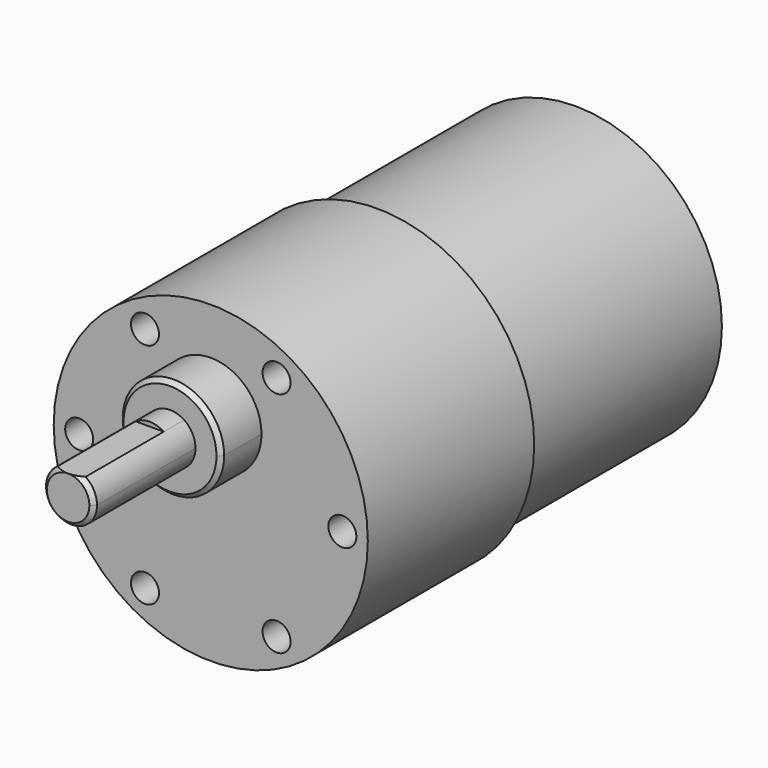
from build123d import *

# Parameters (mm, degrees)
F0_R      = 18.5
F0_R_2    = 17.25
F0_R_3    = 16.7
F0_R_4    = 4.1
F1_DEPTH  = 24.5
F2_DEPTH  = 53.7
F3_R      = 16.7
F3_R_2    = 4.1
F4_DEPTH  = 1
F5_DEPTH  = 1.2
F7_D      = 3.3
F7_DEPTH  = 4
F7_TIP    = 0.9914200214
F8_DEPTH  = 21
F9_DEPTH  = 6
F11_DEPTH = 12
F13_SIZE  = 0.49999


# Not quite as in the source:
# - a fillet or chamfer is up to 0.001 mm smaller than in the source, because OpenCascade refuses the exact size
# - a feature of the source that left no trace in its solid (it failed there, or was rolled back) is left out
# - a feature names something its author has since deleted; it is built from what else it names


with BuildPart() as f1:
    # F0 (on Front) → F1 (new body)
    with BuildSketch(Plane.XZ):
        Circle(F0_R)
        Circle(F0_R_2, mode=Mode.SUBTRACT)
        Circle(F0_R_2)
        Circle(F0_R_3, mode=Mode.SUBTRACT)
        Circle(F0_R_3)
        Circle(F0_R_4, mode=Mode.SUBTRACT)
        Circle(F0_R_4)
    extrude(amount=-F1_DEPTH)

    # F0 (on Front) → F2 (join)
    with BuildSketch(Plane.XZ):
        Circle(F0_R_2)
        Circle(F0_R_3, mode=Mode.SUBTRACT)
        Circle(F0_R_3)
        Circle(F0_R_4, mode=Mode.SUBTRACT)
        Circle(F0_R_4)
    extrude(amount=-F2_DEPTH)

    # F3 (on face) → F4 (cut)
    with BuildSketch(Plane(origin=(0, 53.7, 0), x_dir=(-1, 0, 0), z_dir=(0, 1, 0))):
        Circle(F3_R)
        Circle(F3_R_2, mode=Mode.SUBTRACT)
    extrude(amount=-F4_DEPTH, mode=Mode.SUBTRACT)

    # F5 (add): a face of the model
    f5_faces = [f1.faces().sort_by_distance(p)[0] for p in [
        (0, 53.7, 0),
    ]]
    extrude(f5_faces, amount=F5_DEPTH)

    # F7
    with Locations(Plane.XZ):
        with Locations((7.75, 13.4233937587), (15.5, 0), (7.75, -13.4233937587), (-7.75, -13.4233937587), (-15.5, 0), (-7.75, 13.4233937587)):
            Hole(F7_D / 2, depth=F7_DEPTH)
            with Locations((0, 0, -(F7_DEPTH + F7_TIP / 2))):  # 118° drill point
                Cone(0, F7_D / 2, F7_TIP, mode=Mode.SUBTRACT)

    # F6 (on face) → F8 (join)
    with BuildSketch(Plane.XZ):
        with BuildLine():
            ThreePointArc((0.5863406929, 4.0578571429), (0, 4.1), (-0.5863406929, 4.0578571429))
            ThreePointArc((-0.5863406929, 4.0578571429), (0, 4), (0.5863406929, 4.0578571429))
        make_face()
        with BuildLine():
            ThreePointArc((-1.6583123952, 9.5), (-2.9434412837, 6.4202126173), (-0.5863406929, 4.0578571429))
            ThreePointArc((-0.5863406929, 4.0578571429), (0, 4.1), (0.5863406929, 4.0578571429))
            ThreePointArc((0.5863406929, 4.0578571429), (2.3193772956, 5.0972417493), (3, 7))
            ThreePointArc((3, 7), (2.6433820369, 8.4186371655), (1.6583123952, 9.5))
            Line((1.6583123952, 9.5), (-1.6583123952, 9.5))
        make_face()
        with BuildLine():
            ThreePointArc((1.6583123952, 9.5), (0, 10), (-1.6583123952, 9.5))
            Line((-1.6583123952, 9.5), (1.6583123952, 9.5))
        make_face()
    extrude(amount=F8_DEPTH)

    # F6 (on face) → F9 (join)
    with BuildSketch(Plane.XZ):
        with BuildLine():
            ThreePointArc((-0.5863406929, 4.0578571429), (-2.2505108877, 3.4271271853), (-3.4906475169, 2.1506696429))
            ThreePointArc((-3.4906475169, 2.1506696429), (0, 1.025), (3.4906475169, 2.1506696429))
            ThreePointArc((3.4906475169, 2.1506696429), (2.2505108877, 3.4271271853), (0.5863406929, 4.0578571429))
            ThreePointArc((0.5863406929, 4.0578571429), (0, 4), (-0.5863406929, 4.0578571429))
        make_face()
        with BuildLine():
            ThreePointArc((3.4906475169, 2.1506696429), (5.3177647519, 4.2756646603), (5.975, 7))
            ThreePointArc((5.975, 7), (-2.7243353397, 12.3177647519), (-3.4906475169, 2.1506696429))
            ThreePointArc((-3.4906475169, 2.1506696429), (-2.2505108877, 3.4271271853), (-0.5863406929, 4.0578571429))
            ThreePointArc((-0.5863406929, 4.0578571429), (-2.9434412837, 6.4202126173), (-1.6583123952, 9.5))
            ThreePointArc((-1.6583123952, 9.5), (0, 10), (1.6583123952, 9.5))
            ThreePointArc((1.6583123952, 9.5), (2.6433820369, 8.4186371655), (3, 7))
            ThreePointArc((3, 7), (2.3193772956, 5.0972417493), (0.5863406929, 4.0578571429))
            ThreePointArc((0.5863406929, 4.0578571429), (2.2505108877, 3.4271271853), (3.4906475169, 2.1506696429))
        make_face()
    extrude(amount=F9_DEPTH)

    # F10 (on face) → F11 (cut)
    with BuildSketch(Plane.XZ.offset(21)):
        with BuildLine():
            ThreePointArc((1.6583123952, 9.5), (0, 10), (-1.6583123952, 9.5))
            Line((-1.6583123952, 9.5), (1.6583123952, 9.5))
        make_face()
    extrude(amount=-F11_DEPTH, mode=Mode.SUBTRACT)

    # F13 (size 0.5 in the source; OpenCascade refuses exactly that, so slightly less here)
    f13_edges = [f1.edges().sort_by_distance(p)[0] for p in [
        (-3.490648, -6, 11.84933),
        (0, -21, 4),
    ]]
    chamfer(f13_edges, length=F13_SIZE)


solid = f1.part
